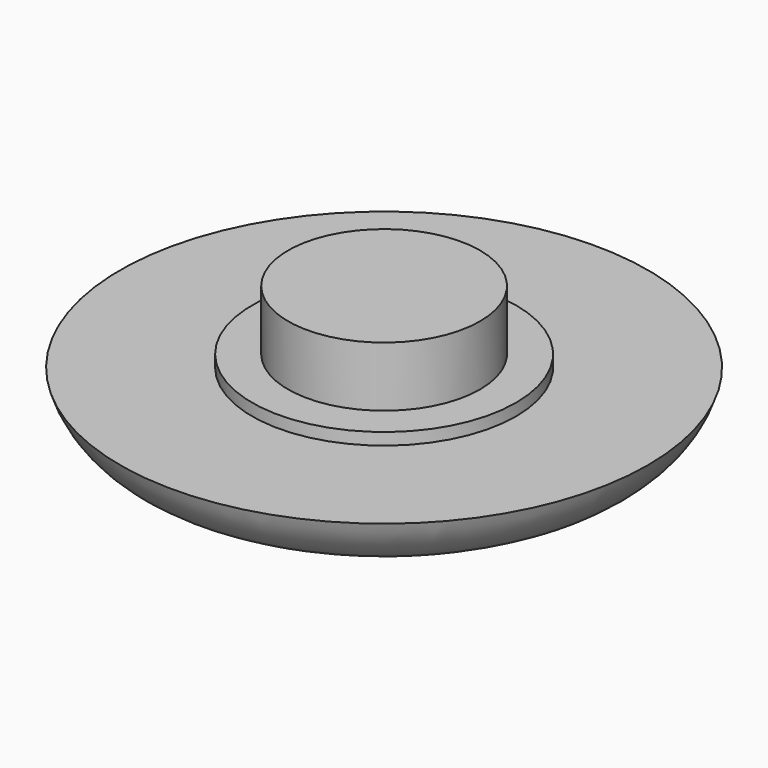
from build123d import *

# Parameters (mm, degrees)
F0_R         = 11
F0_R_2       = 5.5
F1_DEPTH     = 2.5
F0_R_3       = 4
F2_DEPTH     = 3
F3_DEPTH     = 5.5
F6_TEXT_SIZE = 8.7639439023
F7_DEPTH     = 1


# Not quite as in the source:
# - a fillet or chamfer that OpenCascade refuses, or shapes differently, is made with other operations: its cross-section is extruded or revolved along the edge and cut away or added
# - Text() gives the source's letters only with a copy of the font that has no kerning and outlines rounded to 1/6400 em; it was checked with that copy


with BuildPart() as f1:
    # F0 (on Top) → F1 (new body)
    with BuildSketch(Plane.XY):
        Circle(F0_R)
        Circle(F0_R_2, mode=Mode.SUBTRACT)
    extrude(amount=F1_DEPTH)

    # F0 (on Top) → F2 (join, through all)
    with BuildSketch(Plane.XY):
        Circle(F0_R_2)
        Circle(F0_R_3, mode=Mode.SUBTRACT)
    extrude(amount=F2_DEPTH)

    # F0 (on Top) → F3 (join, through all)
    with BuildSketch(Plane.XY):
        Circle(F0_R_3)
    extrude(amount=F3_DEPTH)

    # F4: fillet of radius 3.5 on 1 edges, made by hand

    # F4_s1 → F4_t2 (revolve, cut)
    with BuildSketch(Plane.XZ):
        with BuildLine():
            ThreePointArc((11, 2.5), (9.7375481001, 0.6937569599), (7.6458980338, 0))
            Line((7.6458980338, 0), (11, 0))
            Line((11, 0), (11, 2.5))
        make_face()
    revolve(axis=Axis((0, 0, 0), (0, 0, 1)), mode=Mode.SUBTRACT)

    # F6 (on face) → F7 (cut)
    with BuildSketch(Plane(origin=(0, 0, 0), x_dir=(1, 0, 0), z_dir=(0, 0, -1))):
        with Locations((-6.9645966698, -3.1550198048)):
            Text('D.F', F6_TEXT_SIZE, font='Open Sans', font_style=FontStyle.BOLD, text_align=(TextAlign.LEFT, TextAlign.BOTTOM))
    extrude(amount=-F7_DEPTH, mode=Mode.SUBTRACT)


solid = f1.part
